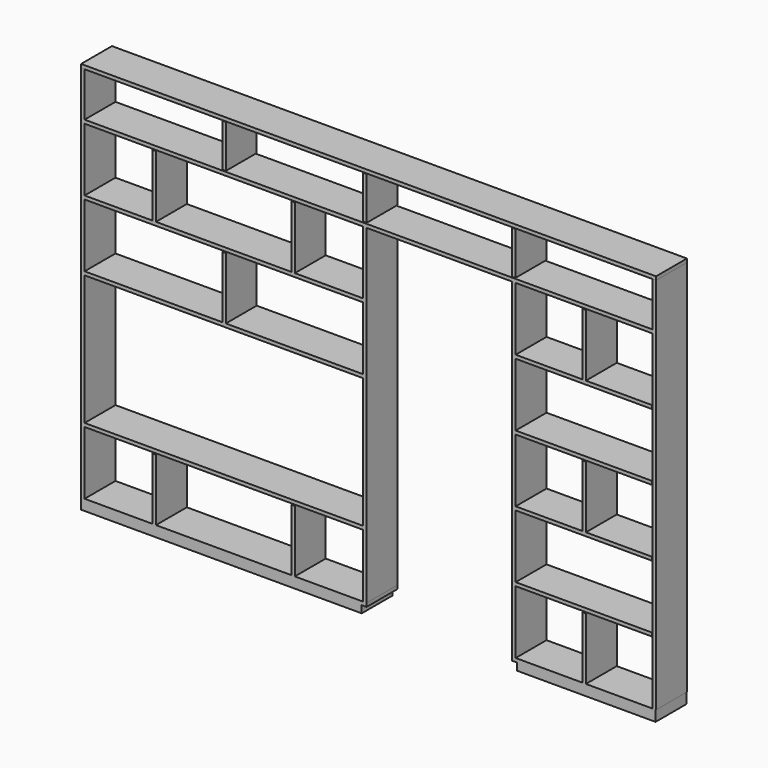
from build123d import *

# Parameters (mm, degrees)
F0_W     = 357.49997
F0_H     = 2.200038
F1_DEPTH = 24
F0_W_2   = 0.000344
F0_W_3   = 2.200038
F0_H_2   = 0.156408
F0_H_3   = 38.543728
F0_H_4   = 38.69359
F0_H_5   = 0.006374
F0_W_4   = 86.200079
F0_H_6   = 0.000344
F0_W_5   = 84.799647
F0_H_7   = 4.499984
F0_W_6   = 174.499943
F0_W_7   = 173.100028
F0_H_8   = 38.618832
F0_H_9   = 0.081304
F0_H_10  = 38.512034
F0_H_11  = 0.18793
F0_H_12  = 26.76822


with BuildPart() as f1:
    # F0 (on Front) → F1 (new body)
    with BuildSketch(Plane.XZ):
        with Locations((0, 120.900114)):
            Rectangle(F0_W, F0_H)
    extrude(amount=F1_DEPTH)


with BuildPart() as f1b:
    # F0 (on Front) → F1, piece 2 (new body)
    with BuildSketch(Plane.XZ):
        Polygon((91.450232, 89.999847), (176.549947, 89.999847), (176.549947, 92.199885), (-176.549947, 92.199885), (-176.549947, 89.999847), (-3.449919, 89.999847), (-1.249881, 89.999847), (89.250194, 89.999847), align=None)
        Polygon((176.549947, 92.199885), (176.549947, 89.999847), (176.549947, -115.300111), (178.450262, -115.300111), (178.749985, -115.300111), (178.749985, 119.79975), (176.549947, 119.79975), align=None)
        Polygon((91.450232, 50.69992), (91.450232, 89.999847), (89.250194, 89.999847), (89.250194, -115.300111), (91.450232, -115.300111), (91.450232, -76.000185), (91.449888, -76.000185), (91.449888, -73.800147), (91.450232, -73.800147), (91.450232, -34.50022), (91.449888, -34.50022), (91.449888, -32.300182), (91.450232, -32.300182), (91.450232, 6.999917), (91.449888, 6.999917), (91.449888, 9.199955), (91.450232, 9.199955), (91.450232, 48.499882), (91.449888, 48.499882), (91.449888, 50.69992), align=None)
        Polygon((178.450262, -115.300111), (176.549947, -115.300111), (135.122674, -115.300111), (135.122674, -115.456519), (132.922636, -115.456519), (132.922636, -115.300111), (91.450232, -115.300111), (89.250194, -115.300111), (89.250194, -117.500149), (92.250183, -117.500149), (92.250183, -117.499805), (178.450262, -117.499805), align=None)
        with Locations((91.45006, 49.599901)):
            Rectangle(F0_W_2, F0_H)
        Polygon((132.922636, 50.69992), (91.450232, 50.69992), (91.450232, 48.499882), (176.249879, 48.499882), (176.249879, 50.69992), (135.122674, 50.69992), (135.122674, 50.693546), (132.922636, 50.693546), align=None)
        Polygon((-176.549947, 89.999847), (-176.549947, 92.199885), (-176.549947, 119.79975), (-178.749985, 119.79975), (-178.749985, -115.300111), (-176.549947, -115.300111), (-176.549947, -76.000185), (-176.549947, -73.800147), (-176.549947, 6.999917), (-176.549947, 9.199955), (-176.549947, 48.499882), (-176.549947, 50.69992), align=None)
        with Locations((134.022655, -115.378315)):
            Rectangle(F0_W_3, F0_H_2)
        with Locations((134.022655, -96.028247)):
            Rectangle(F0_W_3, F0_H_3)
        Polygon((-1.249881, -115.300111), (-1.249881, 89.999847), (-3.449919, 89.999847), (-3.449919, 50.69992), (-3.449919, 48.499882), (-3.449919, 9.199955), (-3.449919, 6.999917), (-3.449919, -73.800147), (-3.449919, -76.000185), (-3.449919, -115.300111), (-1.250053, -115.300111), align=None)
        with Locations((134.022655, 70.046715)):
            Rectangle(F0_W_3, F0_H_4)
        with Locations((134.022655, 50.696733)):
            Rectangle(F0_W_3, F0_H_5)
        with Locations((135.3502225, -117.499977)):
            Rectangle(F0_W_4, F0_H_6)
        with Locations((91.45006, 8.099936)):
            Rectangle(F0_W_2, F0_H)
        with Locations((133.8500555, 8.099936)):
            Rectangle(F0_W_5, F0_H)
        Polygon((-134.393519, 50.69992), (-176.549947, 50.69992), (-176.549947, 48.499882), (-3.449919, 48.499882), (-3.449919, 50.69992), (-45.843369, 50.69992), (-45.843369, 50.693546), (-48.043407, 50.693546), (-48.043407, 50.69992), (-132.193481, 50.69992), (-132.193481, 50.693546), (-134.393519, 50.693546), align=None)
        with Locations((135.3502225, -119.750141)):
            Rectangle(F0_W_4, F0_H_7)
        Polygon((-1.250053, -117.500149), (-1.250053, -115.300111), (-3.449919, -115.300111), (-45.843369, -115.300111), (-45.843369, -115.456519), (-48.043407, -115.456519), (-48.043407, -115.300111), (-132.193481, -115.300111), (-132.193481, -115.456519), (-134.393519, -115.456519), (-134.393519, -115.300111), (-176.549947, -115.300111), (-178.749985, -115.300111), (-178.749985, -117.499805), (-4.250042, -117.499805), (-4.250042, -117.500149), align=None)
        with Locations((133.8500555, -74.900166)):
            Rectangle(F0_W_5, F0_H)
        with Locations((91.45006, -74.900166)):
            Rectangle(F0_W_2, F0_H)
        with Locations((-133.2935, 70.046715)):
            Rectangle(F0_W_3, F0_H_4)
        with Locations((-133.2935, 50.696733)):
            Rectangle(F0_W_3, F0_H_5)
        with Locations((-46.943388, 50.696733)):
            Rectangle(F0_W_3, F0_H_5)
        with Locations((-46.943388, 70.046715)):
            Rectangle(F0_W_3, F0_H_4)
        with Locations((91.45006, -33.400201)):
            Rectangle(F0_W_2, F0_H)
        Polygon((132.922636, -32.300182), (91.450232, -32.300182), (91.450232, -34.50022), (176.249879, -34.50022), (176.249879, -32.300182), (135.122674, -32.300182), (135.122674, -32.381486), (132.922636, -32.381486), align=None)
        Polygon((-90.936396, 9.199955), (-176.549947, 9.199955), (-176.549947, 6.999917), (-3.449919, 6.999917), (-3.449919, 9.199955), (-88.736358, 9.199955), (-88.736358, 9.012025), (-90.936396, 9.012025), align=None)
        with Locations((-91.5000135, -117.499977)):
            Rectangle(F0_W_6, F0_H_6)
        with Locations((-46.943388, -115.378315)):
            Rectangle(F0_W_3, F0_H_2)
        with Locations((-46.943388, -96.028247)):
            Rectangle(F0_W_3, F0_H_3)
        with Locations((-89.999933, -74.900166)):
            Rectangle(F0_W_7, F0_H)
        with Locations((-91.5000135, -119.750141)):
            Rectangle(F0_W_6, F0_H_7)
        with Locations((134.022655, -12.990766)):
            Rectangle(F0_W_3, F0_H_8)
        with Locations((134.022655, -32.340834)):
            Rectangle(F0_W_3, F0_H_9)
        with Locations((-89.836377, 28.455972)):
            Rectangle(F0_W_3, F0_H_10)
        with Locations((-89.836377, 9.10599)):
            Rectangle(F0_W_3, F0_H_11)
        with Locations((-133.2935, -96.028247)):
            Rectangle(F0_W_3, F0_H_3)
        with Locations((-133.2935, -115.378315)):
            Rectangle(F0_W_3, F0_H_2)
    extrude(amount=F1_DEPTH)


with BuildPart() as f1c:
    # F0 (on Front) → F1, piece 3 (new body)
    with BuildSketch(Plane.XZ):
        with Locations((-89.836377, 106.088701)):
            Rectangle(F0_W_3, F0_H_12)
    extrude(amount=F1_DEPTH)


with BuildPart() as f1d:
    # F0 (on Front) → F1, piece 4 (new body)
    with BuildSketch(Plane.XZ):
        with Locations((-2.347488, 106.088701)):
            Rectangle(F0_W_3, F0_H_12)
    extrude(amount=F1_DEPTH)


with BuildPart() as f1e:
    # F0 (on Front) → F1, piece 5 (new body)
    with BuildSketch(Plane.XZ):
        with Locations((90.251683, 106.088701)):
            Rectangle(F0_W_3, F0_H_12)
    extrude(amount=F1_DEPTH)


solid = Compound([f1.part, f1b.part, f1c.part, f1d.part, f1e.part])
